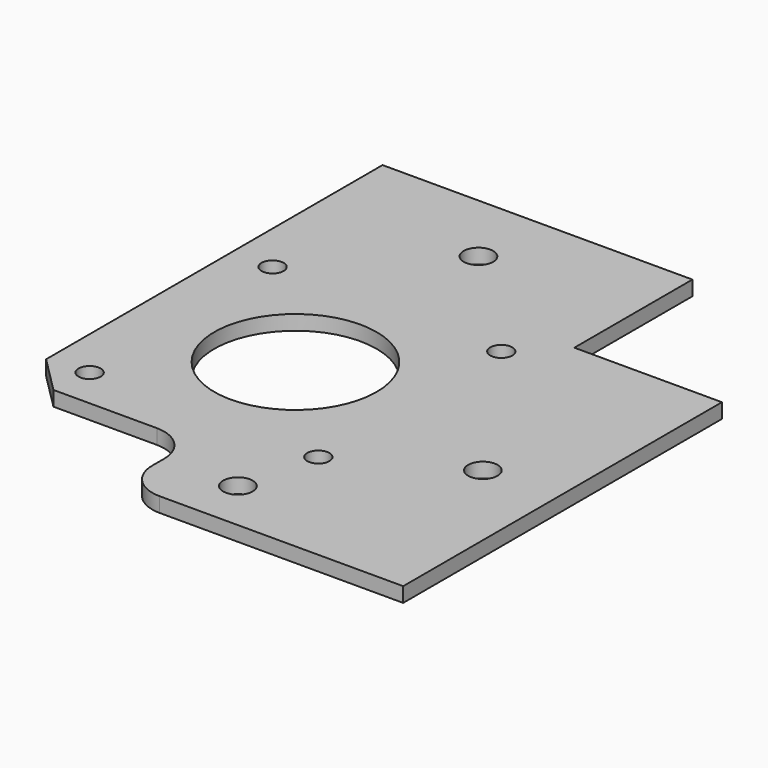
from build123d import *

# Parameters (mm, degrees)
F0_R     = 1.5
F0_R_2   = 11
F0_R_3   = 2
F1_DEPTH = 2
F2_SIZE  = 5
F3_W     = 38
F3_H     = 12
F4_DEPTH = 2
F5_R     = 2
F6_DEPTH = 25
F7_R     = 5


with BuildPart() as f1:
    # F0 (on Top) → F1 (new body)
    with BuildSketch(Plane.XY):
        Polygon((-31, -31), (31, -31), (31, 11), (11, 11), (11, 31), (-31, 31), align=None)
        with Locations((-25.5, -25.5)):
            Circle(F0_R, mode=Mode.SUBTRACT)
        with Locations((-10, -10)):
            Circle(F0_R_2, mode=Mode.SUBTRACT)
        with Locations((5.5, -25.5)):
            Circle(F0_R, mode=Mode.SUBTRACT)
        with Locations((21, -17)):
            Circle(F0_R_3, mode=Mode.SUBTRACT)
        with Locations((-25.5, 5.5)):
            Circle(F0_R, mode=Mode.SUBTRACT)
        with Locations((-10, 21)):
            Circle(F0_R_3, mode=Mode.SUBTRACT)
        with Locations((5.5, 5.5)):
            Circle(F0_R, mode=Mode.SUBTRACT)
    extrude(amount=F1_DEPTH)

    # F2
    f2_edges = [f1.edges().sort_by_distance(p)[0] for p in [
        (-31, -31, 1),
    ]]
    chamfer(f2_edges, length=F2_SIZE)

    # F3 (on face) → F4 (join)
    with BuildSketch(Plane.XY.offset(2)):
        with Locations((12, -37)):
            Rectangle(F3_W, F3_H)
    extrude(amount=-F4_DEPTH)

    # F5 (on face) → F6 (cut)
    with BuildSketch(Plane.XY.offset(2)):
        with Locations((3, -36)):
            Circle(F5_R)
    extrude(amount=-F6_DEPTH, mode=Mode.SUBTRACT)

    # F7
    f7_edges = [f1.edges().sort_by_distance(p)[0] for p in [
        (-7, -43, 1),
        (-7, -31, 1),
    ]]
    fillet(f7_edges, radius=F7_R)


solid = f1.part
